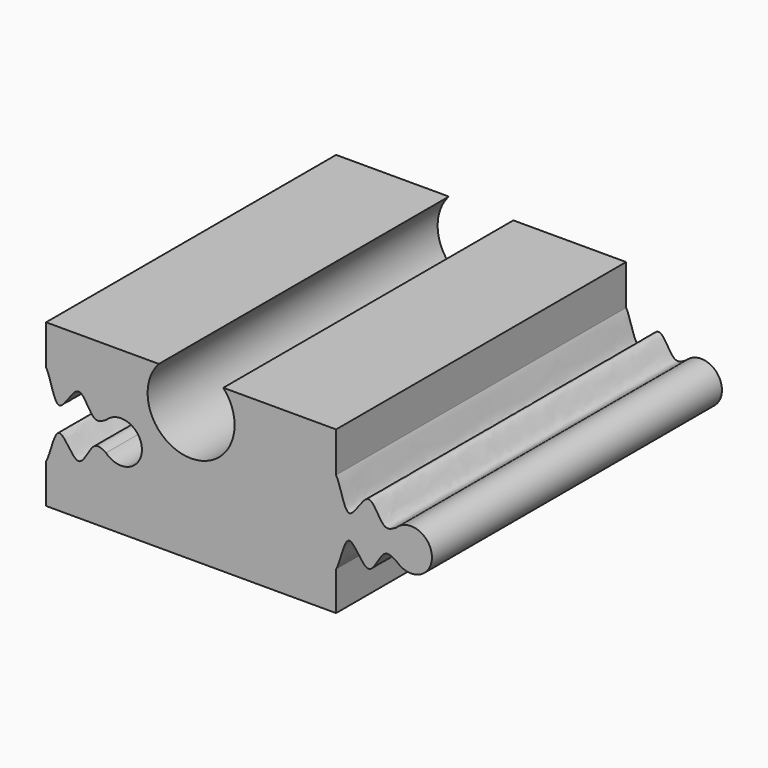
from build123d import *

# Parameters (mm, degrees)
F1_DEPTH = 25


# Not quite as in the source:
# - a feature names something its author has since deleted; it is built from what else it names


with BuildPart() as f1:
    # F0 (on Front) → F1 (new body)
    with BuildSketch(Plane.XZ):
        with BuildLine():
            Line((-10, -5.576437097), (10, -5.576437097))
            Line((10, -5.576437097), (10, -2.9008686543))
            Line((10, -2.9008686543), (10, 2.8053802234))
            Line((10, 2.8053802234), (10, 5.576437097))
            Line((10, 5.576437097), (2.2236531144, 5.576437097))
            ThreePointArc((2.2236531144, 5.576437097), (2.7991926821, 4.6417723907), (3, 3.5626429599))
            ThreePointArc((3, 3.5626429599), (-1.0791294308, 0.7634502778), (-2.2236531144, 5.576437097))
            Line((-2.2236531144, 5.576437097), (-10, 5.576437097))
            Line((-10, 5.576437097), (-10, 2.8429715894))
            add(Edge.make_bspline(
                [(-10, 2.8429715894), (-9.6726290682, 2.2880315783), (-9.2803732694, -0.5143018538), (-7.7135602713, 3.2410752536), (-6.8171719693, 0.3419893756), (-6.0825825554, 0.8733254219), (-5.864968989, 0.9871294023)],
                knots=[0, 0, 0, 0, 0.2957765774, 0.5629842376, 0.8221868806, 1, 1, 1, 1], degree=3))
            ThreePointArc((-5.864968989, 0.9871294023), (-3.3903316246, -0.0101528494), (-5.864968989, -1.0074351012))
            add(Edge.make_bspline(
                [(-10, -2.8632772883), (-9.6726290682, -2.3083372772), (-9.2803732694, 0.4939961549), (-7.7135602713, -3.2613809525), (-6.8171719693, -0.3622950744), (-6.0825825554, -0.8936311207), (-5.864968989, -1.0074351012)],
                knots=[0, 0, 0, 0, 0.2957765774, 0.5629842376, 0.8221868806, 1, 1, 1, 1], degree=3))
            Line((-10, -2.8632772883), (-10, -5.576437097))
        make_face()
        with BuildLine():
            Line((10, 2.8053802234), (10, -2.9008686543))
            add(Edge.make_bspline(
                [(10, -2.9008686543), (10.3273709318, -2.3459286431), (10.7196267306, 0.4564047889), (12.2864397287, -3.2989723184), (13.1828280307, -0.3998864404), (13.9174174446, -0.9312224867), (14.135031011, -1.0450264672)],
                knots=[0, 0, 0, 0, 0.2957765774, 0.5629842376, 0.8221868806, 1, 1, 1, 1], degree=3))
            ThreePointArc((14.135031011, -1.0450264672), (16.6096683754, -0.0477442154), (14.135031011, 0.9495380364))
            add(Edge.make_bspline(
                [(10, 2.8053802234), (10.3273709318, 2.2504402123), (10.7196267306, -0.5518932198), (12.2864397287, 3.2034838876), (13.1828280307, 0.3043980096), (13.9174174446, 0.8357340559), (14.135031011, 0.9495380364)],
                knots=[0, 0, 0, 0, 0.2957765774, 0.5629842376, 0.8221868806, 1, 1, 1, 1], degree=3))
        make_face()
    extrude(amount=F1_DEPTH)


solid = f1.part
